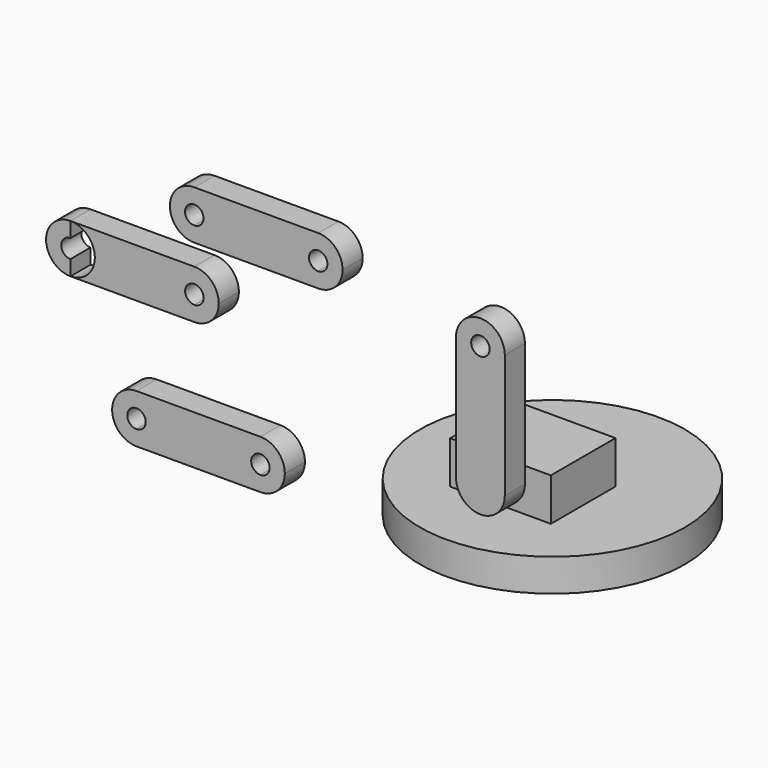
from build123d import *

# Parameters (mm, degrees)
F1_DEPTH = 25.4
F2_R     = 133.9090353396
F3_DEPTH = 32.8763
F4_W     = 101.6
F4_H     = 81.5856331369
F5_DEPTH = 43.0923
F7_DEPTH = 25.4


with BuildPart() as f1:
    # F0 (on Front) → F1 (new body)
    with BuildSketch(Plane.XZ):
        with BuildLine():
            ThreePointArc((-375.1689102501, -33.7191261351), (-382.3788868172, -16.3127029223), (-399.78531003, -9.1027263552))
            Line((-399.78531003, -9.1027263552), (-399.78531003, -24.3999422365))
            ThreePointArc((-399.78531003, -24.3999422365), (-393.1956519002, -27.1294680053), (-390.4661261314, -33.7191261351))
            ThreePointArc((-390.4661261314, -33.7191261351), (-393.1956519002, -40.3087842649), (-399.78531003, -43.0383100337))
            Line((-399.78531003, -43.0383100337), (-399.78531003, -58.335525915))
            ThreePointArc((-399.78531003, -58.335525915), (-382.3788868172, -51.1255493479), (-375.1689102501, -33.7191261351))
        make_face()
        with BuildLine():
            Line((-274.6042609215, -9.1027263552), (-399.78531003, -9.1027263552))
            ThreePointArc((-399.78531003, -9.1027263552), (-382.3788868172, -16.3127029223), (-375.1689102501, -33.7191261351))
            ThreePointArc((-375.1689102501, -33.7191261351), (-382.3788868172, -51.1255493479), (-399.78531003, -58.335525915))
            Line((-399.78531003, -58.335525915), (-274.6042609215, -58.335525915))
            ThreePointArc((-274.6042609215, -58.335525915), (-299.2206607014, -33.7191261351), (-274.6042609215, -9.1027263552))
        make_face()
        with BuildLine():
            Line((-399.78531003, -24.3999422365), (-399.78531003, -9.1027263552))
            ThreePointArc((-399.78531003, -9.1027263552), (-424.4017098099, -33.7191261351), (-399.78531003, -58.335525915))
            Line((-399.78531003, -58.335525915), (-399.78531003, -43.0383100337))
            ThreePointArc((-399.78531003, -43.0383100337), (-409.1044939286, -33.7191261351), (-399.78531003, -24.3999422365))
        make_face()
        with BuildLine():
            ThreePointArc((-249.9878611416, -33.7191261351), (-257.1978377087, -16.3127029223), (-274.6042609215, -9.1027263552))
            Line((-274.6042609215, -9.1027263552), (-274.6042609215, -24.3999422365))
            ThreePointArc((-274.6042609215, -24.3999422365), (-268.0146027917, -27.1294680053), (-265.2850770229, -33.7191261351))
            ThreePointArc((-265.2850770229, -33.7191261351), (-268.0146027917, -40.3087842649), (-274.6042609215, -43.0383100337))
            Line((-274.6042609215, -43.0383100337), (-274.6042609215, -58.335525915))
            ThreePointArc((-274.6042609215, -58.335525915), (-257.1978377087, -51.1255493479), (-249.9878611416, -33.7191261351))
        make_face()
        with BuildLine():
            Line((-274.6042609215, -24.3999422365), (-274.6042609215, -9.1027263552))
            ThreePointArc((-274.6042609215, -9.1027263552), (-299.2206607014, -33.7191261351), (-274.6042609215, -58.335525915))
            Line((-274.6042609215, -58.335525915), (-274.6042609215, -43.0383100337))
            ThreePointArc((-274.6042609215, -43.0383100337), (-283.9234448201, -33.7191261351), (-274.6042609215, -24.3999422365))
        make_face()
    extrude(amount=F1_DEPTH)


with BuildPart() as f1b:
    # F0 (on Front) → F1, piece 2 (new body)
    with BuildSketch(Plane.XZ):
        with BuildLine():
            Line((-341.3049131632, 120.4251348972), (-466.4859622717, 120.4251348972))
            ThreePointArc((-466.4859622717, 120.4251348972), (-449.0795390589, 113.2151583301), (-441.8695624918, 95.8087351173))
            ThreePointArc((-441.8695624918, 95.8087351173), (-449.0795390589, 78.4023119045), (-466.4859622717, 71.1923353374))
            Line((-466.4859622717, 71.1923353374), (-341.3049131632, 71.1923353374))
            ThreePointArc((-341.3049131632, 71.1923353374), (-365.9213129431, 95.8087351173), (-341.3049131632, 120.4251348972))
        make_face()
        with BuildLine():
            ThreePointArc((-316.6885133833, 95.8087351173), (-323.8984899504, 113.2151583301), (-341.3049131632, 120.4251348972))
            Line((-341.3049131632, 120.4251348972), (-341.3049131632, 105.1279190159))
            ThreePointArc((-341.3049131632, 105.1279190159), (-334.7152550334, 102.3983932471), (-331.9857292646, 95.8087351173))
            ThreePointArc((-331.9857292646, 95.8087351173), (-334.7152550334, 89.2190769875), (-341.3049131632, 86.4895512187))
            Line((-341.3049131632, 86.4895512187), (-341.3049131632, 71.1923353374))
            ThreePointArc((-341.3049131632, 71.1923353374), (-323.8984899504, 78.4023119045), (-316.6885133833, 95.8087351173))
        make_face()
        with BuildLine():
            Line((-341.3049131632, 105.1279190159), (-341.3049131632, 120.4251348972))
            ThreePointArc((-341.3049131632, 120.4251348972), (-365.9213129431, 95.8087351173), (-341.3049131632, 71.1923353374))
            Line((-341.3049131632, 71.1923353374), (-341.3049131632, 86.4895512187))
            ThreePointArc((-341.3049131632, 86.4895512187), (-350.6240970618, 95.8087351173), (-341.3049131632, 105.1279190159))
        make_face()
    extrude(amount=F1_DEPTH)


with BuildPart() as f1c:
    # F0 (on Front) → F1, piece 3 (new body)
    with BuildSketch(Plane.XZ):
        with BuildLine():
            Line((-466.4859622717, 105.1279190159), (-466.4859622717, 120.4251348972))
            ThreePointArc((-466.4859622717, 120.4251348972), (-491.1023620516, 95.8087351173), (-466.4859622717, 71.1923353374))
            Line((-466.4859622717, 71.1923353374), (-466.4859622717, 86.4895512187))
            ThreePointArc((-466.4859622717, 86.4895512187), (-475.8051461703, 95.8087351173), (-466.4859622717, 105.1279190159))
        make_face()
    extrude(amount=F1_DEPTH)


with BuildPart() as f3:
    # F2 (on Top) → F3 (new body)
    with BuildSketch(Plane.XY):
        Circle(F2_R)
    extrude(amount=F3_DEPTH)

    # F4 (on face) → F5 (join)
    with BuildSketch(Plane.XY.offset(32.8763)):
        with Locations((-3.2890904695, -20.6068744883)):
            Rectangle(F4_W, F4_H)
    extrude(amount=F5_DEPTH)

    # F6 (on face) → F7, piece 2 (join)
    with BuildSketch(Plane.XZ.offset(61.3996910568)):
        with BuildLine():
            Line((6.0327095305, 184.8320817577), (21.3235095305, 184.8320817577))
            ThreePointArc((21.3235095305, 184.8320817577), (-3.2890904695, 209.4446817577), (-27.9016904695, 184.8320817577))
            Line((-27.9016904695, 184.8320817577), (-12.6108904695, 184.8320817577))
            ThreePointArc((-12.6108904695, 184.8320817577), (-3.2890904695, 194.1538817577), (6.0327095305, 184.8320817577))
        make_face()
        with BuildLine():
            ThreePointArc((-27.9016904695, 184.8320817577), (-3.2890904695, 160.2194817577), (21.3235095305, 184.8320817577))
            Line((21.3235095305, 184.8320817577), (6.0327095305, 184.8320817577))
            ThreePointArc((6.0327095305, 184.8320817577), (-3.2890904695, 175.5102817577), (-12.6108904695, 184.8320817577))
            Line((-12.6108904695, 184.8320817577), (-27.9016904695, 184.8320817577))
        make_face()
        with BuildLine():
            Line((-21.7237969898, 75.9686), (15.1456160509, 75.9686))
            ThreePointArc((15.1456160509, 75.9686), (-3.2890904695, 84.2734817577), (-21.7237969898, 75.9686))
        make_face()
        with BuildLine():
            Line((-27.9016904695, 75.9686), (-27.9016904695, 59.6608817577))
            ThreePointArc((-27.9016904695, 59.6608817577), (-26.3054556958, 68.3802286673), (-21.7237969898, 75.9686))
            Line((-21.7237969898, 75.9686), (-27.9016904695, 75.9686))
        make_face()
        with BuildLine():
            ThreePointArc((15.1456160509, 75.9686), (19.7272747568, 68.3802286673), (21.3235095305, 59.6608817577))
            Line((21.3235095305, 59.6608817577), (21.3235095305, 75.9686))
            Line((21.3235095305, 75.9686), (15.1456160509, 75.9686))
        make_face()
        with BuildLine():
            ThreePointArc((-12.6108904695, 59.6608817577), (-3.2890904695, 68.9826817577), (6.0327095305, 59.6608817577))
            Line((6.0327095305, 59.6608817577), (21.3235095305, 59.6608817577))
            ThreePointArc((21.3235095305, 59.6608817577), (19.7272747568, 68.3802286673), (15.1456160509, 75.9686))
            Line((15.1456160509, 75.9686), (-21.7237969898, 75.9686))
            ThreePointArc((-21.7237969898, 75.9686), (-26.3054556958, 68.3802286673), (-27.9016904695, 59.6608817577))
            Line((-27.9016904695, 59.6608817577), (-12.6108904695, 59.6608817577))
        make_face()
        with BuildLine():
            Line((15.1456160509, 75.9686), (21.3235095305, 75.9686))
            Line((21.3235095305, 75.9686), (21.3235095305, 184.8320817577))
            ThreePointArc((21.3235095305, 184.8320817577), (-3.2890904695, 160.2194817577), (-27.9016904695, 184.8320817577))
            Line((-27.9016904695, 184.8320817577), (-27.9016904695, 75.9686))
            Line((-27.9016904695, 75.9686), (-21.7237969898, 75.9686))
            ThreePointArc((-21.7237969898, 75.9686), (-3.2890904695, 84.2734817577), (15.1456160509, 75.9686))
        make_face()
        with BuildLine():
            Line((21.3235095305, 59.6608817577), (6.0327095305, 59.6608817577))
            ThreePointArc((6.0327095305, 59.6608817577), (-3.2890904695, 50.3390817577), (-12.6108904695, 59.6608817577))
            Line((-12.6108904695, 59.6608817577), (-27.9016904695, 59.6608817577))
            ThreePointArc((-27.9016904695, 59.6608817577), (-3.2890904695, 35.0482817577), (21.3235095305, 59.6608817577))
        make_face()
        with BuildLine():
            Line((-12.6108904695, 59.6608817577), (6.0327095305, 59.6608817577))
            ThreePointArc((6.0327095305, 59.6608817577), (-3.2890904695, 68.9826817577), (-12.6108904695, 59.6608817577))
        make_face()
        with BuildLine():
            ThreePointArc((-12.6108904695, 59.6608817577), (-3.2890904695, 50.3390817577), (6.0327095305, 59.6608817577))
            Line((6.0327095305, 59.6608817577), (-12.6108904695, 59.6608817577))
        make_face()
    extrude(amount=F7_DEPTH)


with BuildPart() as f7:
    # F6 (on face) → F7 (new body)
    with BuildSketch(Plane.XZ.offset(61.3996910568)):
        with BuildLine():
            ThreePointArc((-292.314581573, 198.0006345385), (-301.6337654716, 207.3198184371), (-292.314581573, 216.6390023357))
            Line((-292.314581573, 216.6390023357), (-292.314581573, 231.936218217))
            ThreePointArc((-292.314581573, 231.936218217), (-316.9309813529, 207.3198184371), (-292.314581573, 182.7034186572))
            Line((-292.314581573, 182.7034186572), (-292.314581573, 198.0006345385))
        make_face()
        with BuildLine():
            Line((-167.1335324645, 231.936218217), (-292.314581573, 231.936218217))
            ThreePointArc((-292.314581573, 231.936218217), (-274.9081583602, 224.7262416499), (-267.6981817931, 207.3198184371))
            ThreePointArc((-267.6981817931, 207.3198184371), (-274.9081583602, 189.9133952243), (-292.314581573, 182.7034186572))
            Line((-292.314581573, 182.7034186572), (-167.1335324645, 182.7034186572))
            ThreePointArc((-167.1335324645, 182.7034186572), (-191.7499322444, 207.3198184371), (-167.1335324645, 231.936218217))
        make_face()
        with BuildLine():
            ThreePointArc((-142.5171326846, 207.3198184371), (-149.7271092517, 224.7262416499), (-167.1335324645, 231.936218217))
            Line((-167.1335324645, 231.936218217), (-167.1335324645, 216.6390023357))
            ThreePointArc((-167.1335324645, 216.6390023357), (-160.5438743347, 213.9094765669), (-157.8143485659, 207.3198184371))
            ThreePointArc((-157.8143485659, 207.3198184371), (-160.5438743347, 200.7301603073), (-167.1335324645, 198.0006345385))
            Line((-167.1335324645, 198.0006345385), (-167.1335324645, 182.7034186572))
            ThreePointArc((-167.1335324645, 182.7034186572), (-149.7271092517, 189.9133952243), (-142.5171326846, 207.3198184371))
        make_face()
        with BuildLine():
            ThreePointArc((-292.314581573, 216.6390023357), (-285.7249234432, 213.9094765669), (-282.9953976744, 207.3198184371))
            ThreePointArc((-282.9953976744, 207.3198184371), (-285.7249234432, 200.7301603073), (-292.314581573, 198.0006345385))
            Line((-292.314581573, 198.0006345385), (-292.314581573, 182.7034186572))
            ThreePointArc((-292.314581573, 182.7034186572), (-274.9081583602, 189.9133952243), (-267.6981817931, 207.3198184371))
            ThreePointArc((-267.6981817931, 207.3198184371), (-274.9081583602, 224.7262416499), (-292.314581573, 231.936218217))
            Line((-292.314581573, 231.936218217), (-292.314581573, 216.6390023357))
        make_face()
        with BuildLine():
            Line((-167.1335324645, 216.6390023357), (-167.1335324645, 231.936218217))
            ThreePointArc((-167.1335324645, 231.936218217), (-191.7499322444, 207.3198184371), (-167.1335324645, 182.7034186572))
            Line((-167.1335324645, 182.7034186572), (-167.1335324645, 198.0006345385))
            ThreePointArc((-167.1335324645, 198.0006345385), (-176.4527163631, 207.3198184371), (-167.1335324645, 216.6390023357))
        make_face()
    extrude(amount=F7_DEPTH)


solid = Compound([f1.part, f1b.part, f1c.part, f3.part, f7.part])
